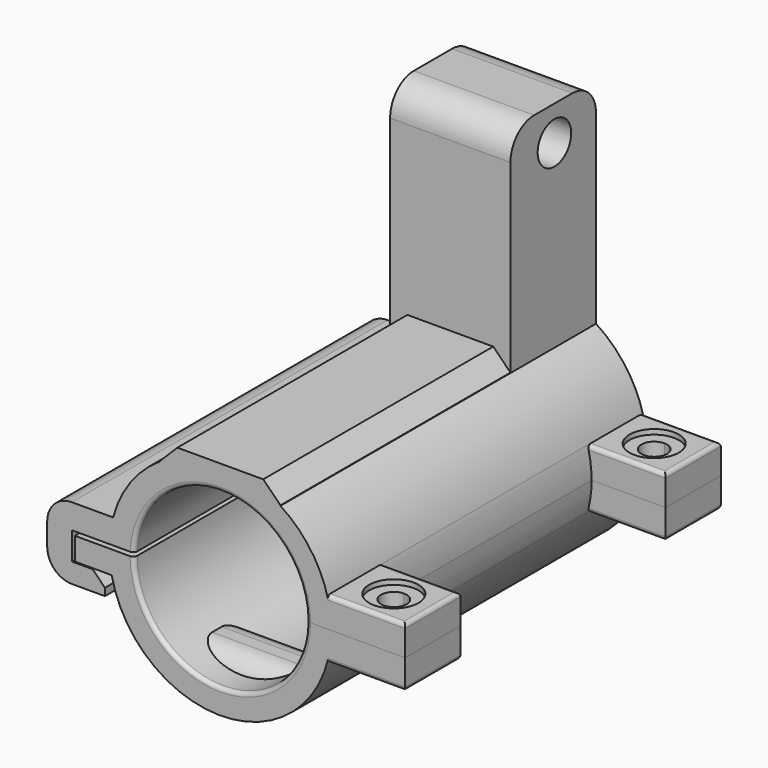
from build123d import *

# Parameters (mm, degrees)
F1_DEPTH      = 80
F2_DEPTH      = 80
F3_START      = 66
F3_DEPTH      = 14
F4_DEPTH      = 14
F5_START      = 66
F5_DEPTH      = 14
F6_DEPTH      = 14
F7_W          = 6
F7_H          = 2.8
F7_H_2        = 2
F8_DEPTH      = 9.5
F8_DEPTH_BACK = 9.5
F9_T4_DEPTH   = 42.9905239528
F9_S5_R       = 17.5
F9_T6_DEPTH   = 23
F9_T10_DEPTH  = 42.9905239528
F9_S11_R      = 17.5
F9_T12_DEPTH  = 23
F9_T16_DEPTH  = 40.2480768093
F9_S17_R      = 17.5
F9_T18_DEPTH  = 22
F9_T22_DEPTH  = 40.2480768093
F9_S23_R      = 17.5
F9_T24_DEPTH  = 22
F12_DEPTH     = 3.8
F13_DEPTH     = 28.501
F15_R         = 5
F15_R_2       = 2.6
F14_R         = 5
F14_R_2       = 2.6
F16_DEPTH     = 1
F17_R         = 5
F18_SIZE      = 2.5
F19_R         = 0.8
F19_2_R       = 0.8
F21_DEPTH     = 80
F22_R         = 4.25
F23_DEPTH     = 49.7010001
F24_SIZE      = 3.5


# Not quite as in the source:
# - a fillet or chamfer that OpenCascade refuses, or shapes differently, is made with other operations: its cross-section is extruded or revolved along the edge and cut away or added
# - a feature names something its author has since deleted; it is built from what else it names


with BuildPart() as f1:
    # F0 (on Front) → F1 (new body)
    with BuildSketch(Plane.XZ):
        with BuildLine():
            ThreePointArc((-22.0247587955, -4.6), (-22.3808743451, -2.3122421047), (-22.5, 0))
            Line((-22.5, 0), (-29.5, 0))
            Line((-29.5, 0), (-29.5, -4.6))
            Line((-29.5, -4.6), (-22.0247587955, -4.6))
        make_face()
        with BuildLine():
            Line((22.5, 0), (17.5, 0))
            ThreePointArc((17.5, 0), (0, -17.5), (-17.5, 0))
            Line((-17.5, 0), (-22.5, 0))
            ThreePointArc((-22.5, 0), (-22.3808743451, -2.3122421047), (-22.0247587955, -4.6))
            ThreePointArc((-22.0247587955, -4.6), (-0.7202894002, -22.488467782), (21.6852484422, -6))
            ThreePointArc((21.6852484422, -6), (22.2953816961, -3.0275328281), (22.5, 0))
        make_face()
    extrude(amount=F1_DEPTH)

    # F0 (on Front) → F5 (join)
    with BuildSketch(Plane.XZ.offset(F5_START)):
        with BuildLine():
            Line((37.5, 0), (22.5, 0))
            ThreePointArc((22.5, 0), (22.2953816961, -3.0275328281), (21.6852484422, -6))
            Line((21.6852484422, -6), (37.5, -6))
            Line((37.5, -6), (37.5, 0))
        make_face()
    extrude(amount=F5_DEPTH)

    # F0 (on Front) → F6 (join)
    with BuildSketch(Plane.XZ):
        with BuildLine():
            Line((37.5, 0), (22.5, 0))
            ThreePointArc((22.5, 0), (22.2953816961, -3.0275328281), (21.6852484422, -6))
            Line((21.6852484422, -6), (37.5, -6))
            Line((37.5, -6), (37.5, 0))
        make_face()
    extrude(amount=F6_DEPTH)

    # F7 (on Right) → F8 (join, two sides)
    with BuildSketch(Plane.YZ) as f8_sk:
        with Locations((-72, -16.1)):
            Rectangle(F7_W, F7_H)
        with Locations((-66, -16.1)):
            Rectangle(F7_W, F7_H)
        with Locations((-14, -16.5)):
            Rectangle(F7_W, F7_H_2)
        with Locations((-8, -16.5)):
            Rectangle(F7_W, F7_H_2)
    extrude(amount=F8_DEPTH)
    extrude(f8_sk.sketch, amount=-F8_DEPTH_BACK)

    # F9: fillet of radius 4.8 on 4 edges, made by hand


with BuildPart() as f2:
    # F0 (on Front) → F2 (new body)
    with BuildSketch(Plane.XZ):
        with BuildLine():
            Line((-30.1, 0.8), (-22.48577328, 0.8))
            ThreePointArc((-22.48577328, 0.8), (-22.2535571218, 3.32102325), (-21.7395952124, 5.8))
            Line((-21.7395952124, 5.8), (-35.1, 5.8))
            Line((-35.1, 5.8), (-35.1, -8.8))
            Line((-35.1, -8.8), (-23.4, -8.8))
            Line((-23.4, -8.8), (-23.4, -4.8))
            Line((-23.4, -4.8), (-30.1, -4.8))
            Line((-30.1, -4.8), (-30.1, 0.8))
        make_face()
        with BuildLine():
            ThreePointArc((-17.4817047224, 0.8), (0.4001045854, 17.4954255827), (17.5, 0))
            Line((17.5, 0), (22.5, 0))
            ThreePointArc((22.5, 0), (22.2953816961, 3.0275328281), (21.6852484422, 6))
            ThreePointArc((21.6852484422, 6), (-0.103626217, 22.4997613678), (-21.7395952124, 5.8))
            ThreePointArc((-21.7395952124, 5.8), (-22.2535571218, 3.32102325), (-22.48577328, 0.8))
            Line((-22.48577328, 0.8), (-17.4817047224, 0.8))
        make_face()
    extrude(amount=F2_DEPTH)

    # F0 (on Front) → F3 (join)
    with BuildSketch(Plane.XZ.offset(F3_START)):
        with BuildLine():
            ThreePointArc((21.6852484422, 6), (22.2953816961, 3.0275328281), (22.5, 0))
            Line((22.5, 0), (37.5, 0))
            Line((37.5, 0), (37.5, 6))
            Line((37.5, 6), (21.6852484422, 6))
        make_face()
    extrude(amount=F3_DEPTH)

    # F0 (on Front) → F4 (join)
    with BuildSketch(Plane.XZ):
        with BuildLine():
            ThreePointArc((21.6852484422, 6), (22.2953816961, 3.0275328281), (22.5, 0))
            Line((22.5, 0), (37.5, 0))
            Line((37.5, 0), (37.5, 6))
            Line((37.5, 6), (21.6852484422, 6))
        make_face()
    extrude(amount=F4_DEPTH)


with BuildPart() as f9_tool2:
    # F9_s3 → F9_t4 (new body)
    with BuildSketch(Plane.YZ.offset(21.4952619764)):
        with BuildLine():
            ThreePointArc((-70.2, -14.7), (-73.5941125497, -16.1058874503), (-75, -19.5))
            Line((-75, -19.5), (-75, -14.7))
            Line((-75, -14.7), (-70.2, -14.7))
        make_face()
    extrude(amount=-F9_T4_DEPTH)

    # F9_s5 → F9_t6 (intersect, symmetric)
    with BuildSketch(Plane.XZ.offset(72.6)):
        Circle(F9_S5_R)
    extrude(amount=F9_T6_DEPTH, both=True, mode=Mode.INTERSECT)


with BuildPart() as f1_1:
    add(f1.part)

    # F9_t1: cut F9_tool2
    add(f9_tool2.part, mode=Mode.SUBTRACT)


with BuildPart() as f9_tool8:
    # F9_s9 → F9_t10 (new body)
    with BuildSketch(Plane.YZ.offset(21.4952619764)):
        with BuildLine():
            ThreePointArc((-63, -19.5), (-64.4058874503, -16.1058874503), (-67.8, -14.7))
            Line((-67.8, -14.7), (-63, -14.7))
            Line((-63, -14.7), (-63, -19.5))
        make_face()
    extrude(amount=-F9_T10_DEPTH)

    # F9_s11 → F9_t12 (intersect, symmetric)
    with BuildSketch(Plane.XZ.offset(65.4)):
        Circle(F9_S11_R)
    extrude(amount=F9_T12_DEPTH, both=True, mode=Mode.INTERSECT)


with BuildPart() as f1_2:
    add(f1_1.part)

    # F9_t7: cut F9_tool8
    add(f9_tool8.part, mode=Mode.SUBTRACT)


with BuildPart() as f9_tool14:
    # F9_s15 → F9_t16 (new body)
    with BuildSketch(Plane.YZ.offset(20.1240384046)):
        with BuildLine():
            ThreePointArc((-17, -20.3), (-15.5941125497, -16.9058874503), (-12.2, -15.5))
            Line((-12.2, -15.5), (-17, -15.5))
            Line((-17, -15.5), (-17, -20.3))
        make_face()
    extrude(amount=-F9_T16_DEPTH)

    # F9_s17 → F9_t18 (intersect, symmetric)
    with BuildSketch(Plane.XZ.offset(14.6)):
        Circle(F9_S17_R)
    extrude(amount=F9_T18_DEPTH, both=True, mode=Mode.INTERSECT)


with BuildPart() as f1_3:
    add(f1_2.part)

    # F9_t13: cut F9_tool14
    add(f9_tool14.part, mode=Mode.SUBTRACT)


with BuildPart() as f9_tool20:
    # F9_s21 → F9_t22 (new body)
    with BuildSketch(Plane.YZ.offset(-20.1240384046)):
        with BuildLine():
            ThreePointArc((-5, -20.3), (-6.4058874503, -16.9058874503), (-9.8, -15.5))
            Line((-9.8, -15.5), (-5, -15.5))
            Line((-5, -15.5), (-5, -20.3))
        make_face()
    extrude(amount=F9_T22_DEPTH)

    # F9_s23 → F9_t24 (intersect, symmetric)
    with BuildSketch(Plane.XZ.offset(7.4)):
        Circle(F9_S23_R)
    extrude(amount=F9_T24_DEPTH, both=True, mode=Mode.INTERSECT)


with BuildPart() as f1_4:
    add(f1_3.part)

    # F9_t19: cut F9_tool20
    add(f9_tool20.part, mode=Mode.SUBTRACT)

    # F10 (on face) + F11 (on face) → F12 (cut)
    with BuildSketch(Plane(origin=(0, 0, -6), x_dir=(1, 0, 0), z_dir=(0, 0, -1))):
        with BuildLine():
            Line((29.6460978174, 78.7732550531), (29.5926242211, 78.7430389296))
            Line((29.5926242211, 78.7430389296), (29.5926242211, 75.6))
            ThreePointArc((29.5926242211, 75.6), (31.4311018522, 74.8384776311), (32.1926242211, 73))
            ThreePointArc((32.1926242211, 73), (31.4311018522, 71.1615223689), (29.5926242211, 70.4))
            Line((29.5926242211, 70.4), (29.5926242211, 67.2569610704))
            Line((29.5926242211, 67.2569610704), (34.5656729615, 70.0670629807))
            Line((34.5656729615, 70.0670629807), (34.6191465577, 75.8403180337))
            Line((34.6191465577, 75.8403180337), (29.6460978174, 78.7732550531))
        make_face()
        with BuildLine():
            Line((29.5926242211, 75.6), (29.5926242211, 78.7430389296))
            Line((29.5926242211, 78.7430389296), (24.6195754807, 75.9329370193))
            Line((24.6195754807, 75.9329370193), (24.5661018845, 70.1596819663))
            Line((24.5661018845, 70.1596819663), (29.5391506248, 67.2267449469))
            Line((29.5391506248, 67.2267449469), (29.5926242211, 67.2569610704))
            Line((29.5926242211, 67.2569610704), (29.5926242211, 70.4))
            ThreePointArc((29.5926242211, 70.4), (26.9926242211, 73), (29.5926242211, 75.6))
        make_face()
    with BuildSketch(Plane(origin=(0, 0, -6), x_dir=(1, 0, 0), z_dir=(0, 0, -1))):
        with BuildLine():
            Line((29.6402919848, 12.7733059089), (29.5926242211, 12.7463071867))
            Line((29.5926242211, 12.7463071867), (29.5926242211, 9.6))
            ThreePointArc((29.5926242211, 9.6), (31.4311018522, 8.8384776311), (32.1926242211, 7))
            ThreePointArc((32.1926242211, 7), (31.4311018522, 5.1615223689), (29.5926242211, 4.4))
            Line((29.5926242211, 4.4), (29.5926242211, 1.2536928133))
            Line((29.5926242211, 1.2536928133), (34.5686199202, 4.0720655513))
            Line((34.5686199202, 4.0720655513), (34.6162876839, 9.8453714602))
            Line((34.6162876839, 9.8453714602), (29.6402919848, 12.7733059089))
        make_face()
        with BuildLine():
            Line((29.5926242211, 9.6), (29.5926242211, 12.7463071867))
            Line((29.5926242211, 12.7463071867), (24.616628522, 9.9279344487))
            Line((24.616628522, 9.9279344487), (24.5689607583, 4.1546285398))
            Line((24.5689607583, 4.1546285398), (29.5449564574, 1.2266940911))
            Line((29.5449564574, 1.2266940911), (29.5926242211, 1.2536928133))
            Line((29.5926242211, 1.2536928133), (29.5926242211, 4.4))
            ThreePointArc((29.5926242211, 4.4), (26.9926242211, 7), (29.5926242211, 9.6))
        make_face()
    extrude(amount=-F12_DEPTH, mode=Mode.SUBTRACT)


with BuildPart() as f13_tool:
    # F13 (cut, through all): faces of the model
    f13_faces = [f1_4.part.faces().sort_by_distance(p)[0] for p in [
        (29.5926242211, -73, -6),
        (29.5926242211, -7, -6),
    ]]
    extrude(f13_faces, amount=-F13_DEPTH)


with BuildPart() as f1_5:
    add(f1_4.part)

    # F13: cut by f13_tool
    add(f13_tool.part, mode=Mode.SUBTRACT)

    # F19
    f19_edges = [f1_5.edges().sort_by_distance(p)[0] for p in [
        (29.592624, -80, -6),
        (37.5, -73, -6),
        (29.592624, -66, -6),
        (29.592624, 0, -6),
        (37.5, -7, -6),
        (29.592624, -14, -6),
        (0, 0, -17.5),
        (0, -80, -17.5),
    ]]
    fillet(f19_edges, radius=F19_R)


with BuildPart() as f2_1:
    add(f2.part)

    # F13: cut by f13_tool
    add(f13_tool.part, mode=Mode.SUBTRACT)

    # F15 (on face) + F14 (on face) → F16 (cut)
    with BuildSketch(Plane.XY.offset(6)):
        with Locations((29.5926242211, -7)):
            Circle(F15_R)
        with Locations((29.5926242211, -7)):
            Circle(F15_R_2, mode=Mode.SUBTRACT)
    with BuildSketch(Plane.XY.offset(6)):
        with Locations((29.5926242211, -73)):
            Circle(F14_R)
        with Locations((29.5926242211, -73)):
            Circle(F14_R_2, mode=Mode.SUBTRACT)
    extrude(amount=-F16_DEPTH, mode=Mode.SUBTRACT)

    # F17
    f17_edges = [f2_1.edges().sort_by_distance(p)[0] for p in [
        (-35.1, -40, 5.8),
        (-35.1, -40, -8.8),
    ]]
    fillet(f17_edges, radius=F17_R)

    # F18
    f18_edges = [f2_1.edges().sort_by_distance(p)[0] for p in [
        (-23.4, -40, -4.8),
    ]]
    chamfer(f18_edges, length=F18_SIZE)

    # F19#2
    f19_2_edges = [f2_1.edges().sort_by_distance(p)[0] for p in [
        (29.592624, -80, 6),
        (37.5, -73, 6),
        (29.592624, -66, 6),
        (29.592624, -14, 6),
        (37.5, -7, 6),
        (29.592624, 0, 6),
        (0.400105, 0, 17.495426),
        (0.400105, -80, 17.495426),
    ]]
    fillet(f19_2_edges, radius=F19_2_R)

    # F20 (on Front) → F21 (join)
    with BuildSketch(Plane.XZ):
        with BuildLine():
            ThreePointArc((-12.2, 18.9052902649), (0, 22.5), (12.2, 18.9052902649))
            Line((12.2, 18.9052902649), (12.2, 62.5))
            Line((12.2, 62.5), (-12.2, 62.5))
            Line((-12.2, 62.5), (-12.2, 18.9052902649))
        make_face()
    extrude(amount=F21_DEPTH)

    # F22 (on face) → F23 (cut, through all)
    with BuildSketch(Plane(origin=(-12.2, 0, 0), x_dir=(0, -1, 0), z_dir=(-1, 0, 0))):
        with Locations((10.5445438474, 55.4783681659)):
            Circle(F22_R)
        with BuildLine():
            Line((0, 62.5), (0, 56.5))
            ThreePointArc((0, 56.5), (1.7573593129, 60.7426406871), (6, 62.5))
            Line((6, 62.5), (0, 62.5))
        make_face()
        with BuildLine():
            Line((21.6961836666, 56.5), (21.6961836666, 22.5))
            Line((21.6961836666, 22.5), (80, 22.5))
            Line((80, 22.5), (80, 62.5))
            Line((80, 62.5), (15.6961836666, 62.5))
            ThreePointArc((15.6961836666, 62.5), (19.9388243537, 60.7426406871), (21.6961836666, 56.5))
        make_face()
    extrude(amount=-F23_DEPTH, mode=Mode.SUBTRACT)

    # F24
    f24_edges = [f2_1.edges().sort_by_distance(p)[0] for p in [
        (-12.2, -50.848092, 22.5),
        (12.2, -50.848092, 22.5),
    ]]
    chamfer(f24_edges, length=F24_SIZE)


solid = Compound([f1_5.part, f2_1.part])
